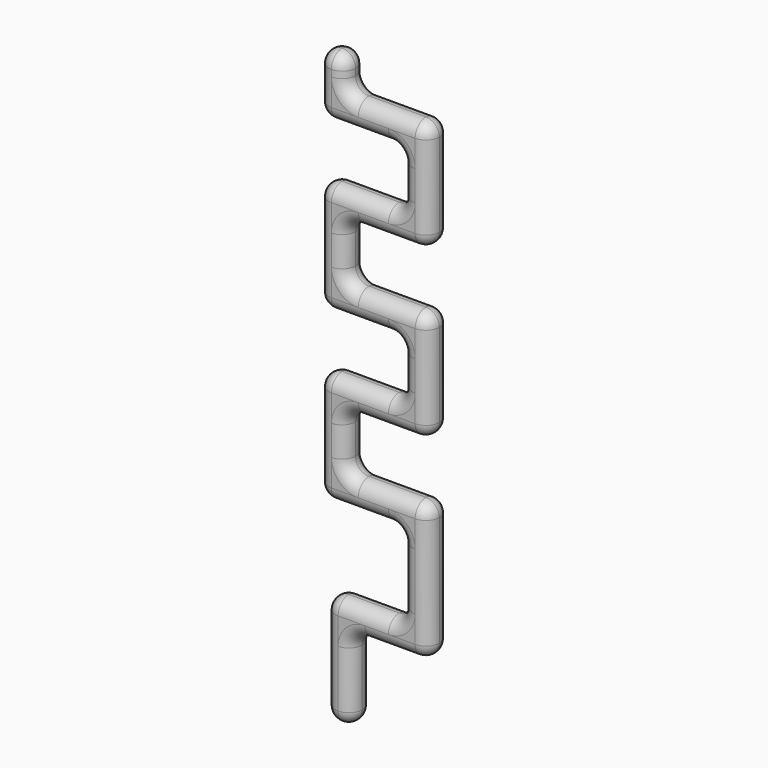
from build123d import *

# Parameters (mm, degrees)
F0_W      = 8
F0_H      = 8
F1_DEPTH  = 33
F2_W      = 8
F2_H      = 8
F3_DEPTH  = 23
F4_W      = 8
F4_H      = 8
F5_DEPTH  = 41
F6_W      = 8
F6_H      = 8
F7_DEPTH  = 25
F8_W      = 8
F8_H      = 8
F9_DEPTH  = 25
F10_W     = 8
F10_H     = 8
F11_DEPTH = 25
F12_W     = 8
F12_H     = 8
F13_DEPTH = 25
F14_W     = 8
F14_H     = 8
F15_DEPTH = 25
F16_W     = 8
F16_H     = 8
F17_DEPTH = 25
F18_W     = 8
F18_H     = 8
F19_DEPTH = 25
F20_W     = 8
F20_H     = 8
F21_DEPTH = 25
F22_W     = 8
F22_H     = 8
F23_DEPTH = 25
F24_W     = 8
F24_H     = 8
F25_DEPTH = 10
F26_R     = 3.99999


# Not quite as in the source:
# - a fillet or chamfer is up to 0.001 mm smaller than in the source, because OpenCascade refuses the exact size


with BuildPart() as f1:
    # F0 (on Top) → F1 (new body)
    with BuildSketch(Plane.XY):
        with Locations((-53.9294078052, -0.6740109101)):
            Rectangle(F0_W, F0_H)
    extrude(amount=F1_DEPTH)

    # F2 (on face) → F3 (join)
    with BuildSketch(Plane.YZ.offset(-49.9294078052)):
        with Locations((-0.6740109101, 29)):
            Rectangle(F2_W, F2_H)
    extrude(amount=F3_DEPTH)

    # F4 (on face) → F5 (join)
    with BuildSketch(Plane(origin=(0, 0, 25), x_dir=(1, 0, 0), z_dir=(0, 0, -1))):
        with Locations((-30.9294078052, 0.6740109101)):
            Rectangle(F4_W, F4_H)
    extrude(amount=-F5_DEPTH)

    # F6 (on face) → F7 (join)
    with BuildSketch(Plane(origin=(-34.9294078052, 0, 0), x_dir=(0, -1, 0), z_dir=(-1, 0, 0))):
        with Locations((0.6740109101, 62)):
            Rectangle(F6_W, F6_H)
    extrude(amount=F7_DEPTH)

    # F8 (on face) → F9 (join)
    with BuildSketch(Plane.XY.offset(66)):
        with Locations((-55.9294078052, -0.6740109101)):
            Rectangle(F8_W, F8_H)
    extrude(amount=F9_DEPTH)

    # F10 (on face) → F11 (join)
    with BuildSketch(Plane.YZ.offset(-51.9294078052)):
        with Locations((-0.6740109101, 87)):
            Rectangle(F10_W, F10_H)
    extrude(amount=F11_DEPTH)

    # F12 (on face) → F13 (join)
    with BuildSketch(Plane.XY.offset(91)):
        with Locations((-30.9294078052, -0.6740109101)):
            Rectangle(F12_W, F12_H)
    extrude(amount=F13_DEPTH)

    # F14 (on face) → F15 (join)
    with BuildSketch(Plane(origin=(-34.9294078052, 0, 0), x_dir=(0, -1, 0), z_dir=(-1, 0, 0))):
        with Locations((0.6740109101, 112)):
            Rectangle(F14_W, F14_H)
    extrude(amount=F15_DEPTH)

    # F16 (on face) → F17 (join)
    with BuildSketch(Plane.XY.offset(116)):
        with Locations((-55.9294078052, -0.6740109101)):
            Rectangle(F16_W, F16_H)
    extrude(amount=F17_DEPTH)

    # F18 (on face) → F19 (join)
    with BuildSketch(Plane.YZ.offset(-51.9294078052)):
        with Locations((-0.6740109101, 137)):
            Rectangle(F18_W, F18_H)
    extrude(amount=F19_DEPTH)

    # F20 (on face) → F21 (join)
    with BuildSketch(Plane.XY.offset(141)):
        with Locations((-30.9294078052, -0.6740109101)):
            Rectangle(F20_W, F20_H)
    extrude(amount=F21_DEPTH)

    # F22 (on face) → F23 (join)
    with BuildSketch(Plane(origin=(-34.9294078052, 0, 0), x_dir=(0, -1, 0), z_dir=(-1, 0, 0))):
        with Locations((0.6740109101, 162)):
            Rectangle(F22_W, F22_H)
    extrude(amount=F23_DEPTH)

    # F24 (on face) → F25 (join)
    with BuildSketch(Plane.XY.offset(166)):
        with Locations((-55.9294078052, -0.6740109101)):
            Rectangle(F24_W, F24_H)
    extrude(amount=F25_DEPTH)

    # F26 (radius 4 in the source; OpenCascade refuses exactly that, so slightly less here)
    f26_edges = [f1.edges().sort_by_distance(p)[0] for p in [
        (-38.429408, 3.325989, 25),
        (-46.429408, -4.674011, 33),
        (-26.929408, -0.674011, 83),
        (-26.929408, 3.325989, 99.5),
        (-26.929408, -0.674011, 116),
        (-26.929408, -4.674011, 99.5),
        (-34.929408, -4.674011, 99.5),
        (-59.929408, 3.325989, 124.5),
        (-59.929408, -0.674011, 108),
        (-59.929408, -4.674011, 124.5),
        (-59.929408, -0.674011, 141),
        (-53.929408, -4.674011, 0),
        (-39.429408, -4.674011, 116),
        (-59.929408, -0.674011, 58),
        (-59.929408, -4.674011, 74.5),
        (-59.929408, -0.674011, 91),
        (-59.929408, 3.325989, 74.5),
        (-47.429408, 3.325989, 58),
        (-47.429408, -4.674011, 58),
        (-34.929408, -0.674011, 58),
        (-51.929408, -4.674011, 171),
        (-51.929408, 3.325989, 171),
        (-47.429408, -4.674011, 91),
        (-26.929408, 3.325989, 149.5),
        (-26.929408, -0.674011, 133),
        (-26.929408, -0.674011, 166),
        (-26.929408, -4.674011, 149.5),
        (-34.929408, -0.674011, 141),
        (-34.929408, -4.674011, 149.5),
        (-34.929408, -0.674011, 158),
        (-34.929408, 3.325989, 149.5),
        (-51.929408, -4.674011, 74.5),
        (-51.929408, -4.674011, 124.5),
        (-34.929408, 3.325989, 45.5),
        (-34.929408, -4.674011, 45.5),
        (-34.929408, -0.674011, 33),
        (-47.429408, -4.674011, 141),
        (-47.429408, -4.674011, 108),
        (-39.429408, -4.674011, 83),
        (-39.429408, 3.325989, 83),
        (-51.929408, -0.674011, 83),
        (-38.429408, -4.674011, 25),
        (-47.429408, 3.325989, 158),
        (-47.429408, -4.674011, 158),
        (-59.929408, -0.674011, 158),
        (-51.929408, -0.674011, 166),
        (-51.929408, -0.674011, 176),
        (-39.429408, 3.325989, 133),
        (-34.929408, -0.674011, 91),
        (-34.929408, -0.674011, 108),
        (-34.929408, 3.325989, 99.5),
        (-26.929408, 3.325989, 45.5),
        (-26.929408, -0.674011, 66),
        (-26.929408, -4.674011, 45.5),
        (-26.929408, -0.674011, 25),
        (-39.429408, -4.674011, 166),
        (-39.429408, 3.325989, 166),
        (-59.929408, -4.674011, 167),
        (-59.929408, -0.674011, 176),
        (-59.929408, 3.325989, 167),
        (-47.429408, 3.325989, 108),
        (-47.429408, 3.325989, 91),
        (-51.929408, -0.674011, 116),
        (-39.429408, 3.325989, 116),
        (-51.929408, 3.325989, 74.5),
        (-39.429408, 3.325989, 66),
        (-51.929408, -0.674011, 66),
        (-39.429408, -4.674011, 66),
        (-39.429408, -4.674011, 133),
        (-51.929408, 3.325989, 124.5),
        (-49.929408, -0.674011, 25),
        (-47.429408, 3.325989, 141),
        (-51.929408, -0.674011, 133),
        (-46.429408, 3.325989, 33),
        (-57.929408, -0.674011, 33),
        (-55.929408, -4.674011, 176),
        (-55.929408, 3.325989, 176),
        (-53.929408, 3.325989, 0),
        (-49.929408, 3.325989, 12.5),
        (-57.929408, 3.325989, 16.5),
        (-57.929408, -4.674011, 16.5),
        (-49.929408, -4.674011, 12.5),
        (-57.929408, -0.674011, 0),
        (-49.929408, -0.674011, 0),
    ]]
    fillet(f26_edges, radius=F26_R)


solid = f1.part
